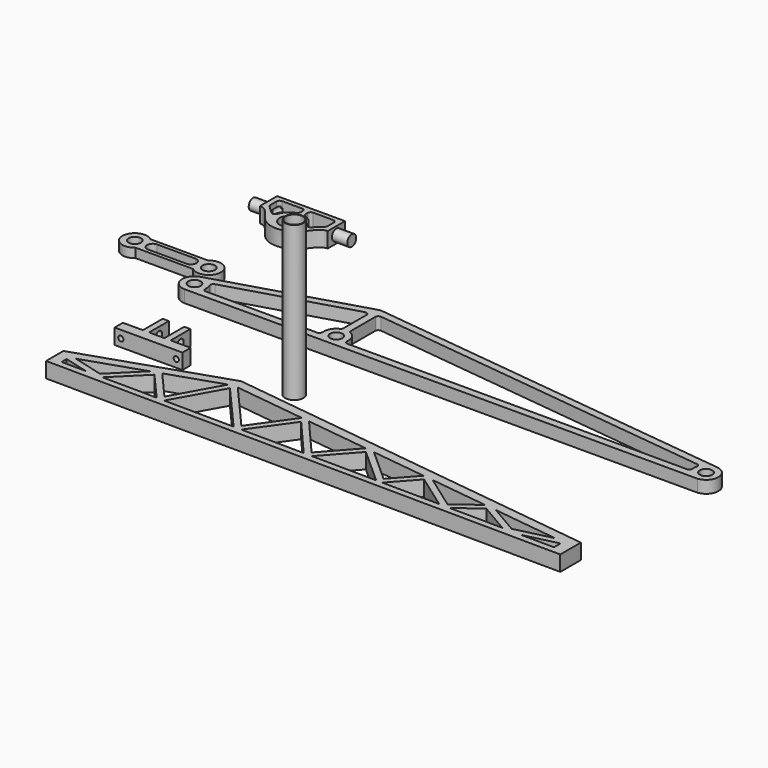
from build123d import *

# Parameters (mm, degrees)
F0_R      = 10
F1_DEPTH  = 20
F2_R      = 5
F3_R      = 10
F4_DEPTH  = 15
F5_R      = 15
F6_DEPTH  = 25
F7_R      = 9
F8_DEPTH  = 25
F13_DEPTH = 25
F14_R     = 6.3615606468
F15_DEPTH = 238.9008327255
F16_R     = 4.25
F17_DEPTH = 16.7239428354
F18_R     = 4.5979762067
F19_DEPTH = 20
F21_R     = 15
F21_R_2   = 14
F22_DEPTH = 250
F24_DEPTH = 25


# Not quite as in the source:
# - a feature of the source that left no trace in its solid (it failed there, or was rolled back) is left out
# - a pattern or mirror of a feature is missing from the dataset's text; its kind, count and spacing are read off the source's solid


with BuildPart() as f1:
    # F0 (on Top) → F1 (new body)
    with BuildSketch(Plane.XY):
        with BuildLine():
            Line((567.1867912898, 20), (-31.031592147, 89.5228215324))
            ThreePointArc((-31.031592147, 89.5228215324), (-35.1003415232, 89.5789443296), (-39.0962379428, 88.81038525))
            Line((-39.0962379428, 88.81038525), (-270.8933937767, 19.1538539919))
            ThreePointArc((-270.8933937767, 19.1538539919), (-284.9248706815, -2.9088588966), (-265.1375378668, -20))
            Line((-265.1375378668, -20), (567.1867912898, -20))
            ThreePointArc((567.1867912898, -20), (584.9970717899, 0), (567.1867912898, 20))
        make_face()
        with Locations((-265.1375378668, 0)):
            Circle(F0_R, mode=Mode.SUBTRACT)
        with Locations((-35.1375378668, 0)):
            Circle(F0_R, mode=Mode.SUBTRACT)
        with BuildLine():
            ThreePointArc((-246.807235087, -8), (-245.3502050521, 2.9088588966), (-249.8850830771, 12.936870676))
            Line((-249.8850830771, 12.936870676), (-41.1375378668, 75.6668461828))
            Line((-41.1375378668, 75.6668461828), (-41.1375378668, 19.0787840283))
            ThreePointArc((-41.1375378668, 19.0787840283), (-53.3393521844, 8.2881816792), (-53.4678406467, -8))
            Line((-53.4678406467, -8), (-246.807235087, -8))
        make_face(mode=Mode.SUBTRACT)
        with Locations((564.8624621332, 0)):
            Circle(F0_R, mode=Mode.SUBTRACT)
        with BuildLine():
            ThreePointArc((-16.807235087, -8), (-16.9357235492, 8.2881816792), (-29.1375378668, 19.0787840283))
            Line((-29.1375378668, 19.0787840283), (-29.1375378668, 77.221935459))
            Line((-29.1375378668, 77.221935459), (547.6527036309, 10.1894166807))
            ThreePointArc((547.6527036309, 10.1894166807), (544.9003052161, 1.2297525035), (546.5321593533, -8))
            Line((546.5321593533, -8), (-16.807235087, -8))
        make_face(mode=Mode.SUBTRACT)
    extrude(amount=F1_DEPTH)

    # F2
    f2_edges = [f1.edges().sort_by_distance(p)[0] for p in [
        (547.652704, 10.189417, 10),
        (546.532159, -8, 10),
        (-29.137538, 77.221935, 10),
        (-29.137538, 19.078784, 10),
        (-16.807235, -8, 10),
        (-53.467841, -8, 10),
        (-41.137538, 19.078784, 10),
        (-41.137538, 75.666846, 10),
        (-246.807235, -8, 10),
        (-249.885083, 12.936871, 10),
    ]]
    fillet(f2_edges, radius=F2_R)


with BuildPart() as f4:
    # F3 (on Top) → F4 (new body)
    with BuildSketch(Plane.XY):
        with BuildLine():
            Line((-297.414090761, 67.674737215), (-390.9565776503, 67.674737215))
            ThreePointArc((-390.9565776503, 67.674737215), (-424.1853342056, 52.674737215), (-390.9565776503, 37.674737215))
            Line((-390.9565776503, 37.674737215), (-297.414090761, 37.674737215))
            ThreePointArc((-297.414090761, 37.674737215), (-264.1853342056, 52.674737215), (-297.414090761, 67.674737215))
        make_face()
        with Locations((-404.1853342056, 52.674737215)):
            Circle(F3_R, mode=Mode.SUBTRACT)
        with Locations((-284.1853342056, 52.674737215)):
            Circle(F3_R, mode=Mode.SUBTRACT)
        with BuildLine():
            ThreePointArc((-375.1853342056, 43.674737215), (-384.1853342056, 52.674737215), (-375.1853342056, 61.674737215))
            Line((-375.1853342056, 61.674737215), (-313.1853342056, 61.674737215))
            ThreePointArc((-313.1853342056, 61.674737215), (-304.1853342056, 52.674737215), (-313.1853342056, 43.674737215))
            Line((-313.1853342056, 43.674737215), (-375.1853342056, 43.674737215))
        make_face(mode=Mode.SUBTRACT)
    extrude(amount=F4_DEPTH)


with BuildPart() as f6:
    # F5 (on Top) → F6 (new body)
    with BuildSketch(Plane.XY):
        with BuildLine():
            Line((-217.3005115986, 245.3892374753), (-327.3005115986, 245.3892374753))
            Line((-327.3005115986, 245.3892374753), (-327.3005115986, 210.3892374753))
            add(Edge.make_bspline(
                [(-327.3005115986, 210.3892374753), (-307.3005115986, 210.3892374753), (-307.3005115986, 175.3892374753), (-272.3005115986, 175.3892374753)],
                knots=[0, 0, 0, 0, 65.192024052, 65.192024052, 65.192024052, 65.192024052], degree=3))
            add(Edge.make_bspline(
                [(-217.3005115986, 210.3892374753), (-237.3005115986, 210.3892374753), (-237.3005115986, 175.3892374753), (-272.3005115986, 175.3892374753)],
                knots=[0, 0, 0, 0, 65.192024052, 65.192024052, 65.192024052, 65.192024052], degree=3))
            Line((-217.3005115986, 210.3892374753), (-217.3005115986, 245.3892374753))
        make_face()
        with Locations((-272.3005115986, 200.3892374753)):
            Circle(F5_R, mode=Mode.SUBTRACT)
        with BuildLine():
            Line((-313.7724625721, 238.4117428172), (-281.3005115986, 238.4117428172))
            ThreePointArc((-281.3005115986, 238.4117428172), (-277.7649776927, 236.9472767232), (-276.3005115986, 233.4117428172))
            Line((-276.3005115986, 233.4117428172), (-276.3005115986, 229.7345567962))
            ThreePointArc((-276.3005115986, 229.7345567962), (-277.4218413879, 226.2407813042), (-280.3669495445, 224.0521320333))
            ThreePointArc((-280.3669495445, 224.0521320333), (-290.3349269514, 217.7028120017), (-296.2725894189, 207.4842698908))
            ThreePointArc((-296.2725894189, 207.4842698908), (-299.7611526365, 204.0768129016), (-304.4918862976, 205.2604494523))
            Line((-304.4918862976, 205.2604494523), (-317.1973438867, 217.2057560035))
            ThreePointArc((-317.1973438867, 217.2057560035), (-318.3618201836, 218.8641946784), (-318.7724625721, 220.848582925))
            Line((-318.7724625721, 220.848582925), (-318.7724625721, 233.4117428172))
            ThreePointArc((-318.7724625721, 233.4117428172), (-317.307996478, 236.9472767232), (-313.7724625721, 238.4117428172))
        make_face(mode=Mode.SUBTRACT)
        with BuildLine():
            ThreePointArc((-248.3284337783, 207.4842698908), (-254.2660962457, 217.7028120017), (-264.2340736527, 224.0521320333))
            ThreePointArc((-264.2340736527, 224.0521320333), (-267.1791818093, 226.2407813042), (-268.3005115986, 229.7345567962))
            Line((-268.3005115986, 229.7345567962), (-268.3005115986, 233.4117428172))
            ThreePointArc((-268.3005115986, 233.4117428172), (-266.8360455045, 236.9472767232), (-263.3005115986, 238.4117428172))
            Line((-263.3005115986, 238.4117428172), (-230.8285606251, 238.4117428172))
            ThreePointArc((-230.8285606251, 238.4117428172), (-227.2930267191, 236.9472767232), (-225.8285606251, 233.4117428172))
            Line((-225.8285606251, 233.4117428172), (-225.8285606251, 220.848582925))
            ThreePointArc((-225.8285606251, 220.848582925), (-226.2392030135, 218.8641946784), (-227.4036793104, 217.2057560035))
            Line((-227.4036793104, 217.2057560035), (-240.1091368996, 205.2604494523))
            ThreePointArc((-240.1091368996, 205.2604494523), (-244.8398705607, 204.0768129016), (-248.3284337783, 207.4842698908))
        make_face(mode=Mode.SUBTRACT)
    extrude(amount=F6_DEPTH)

    # F7 (on face) → F8 (join)
    with BuildSketch(Plane(origin=(-327.3005115986, 0, 0), x_dir=(0, -1, 0), z_dir=(-1, 0, 0))):
        with Locations((-227.8892374753, 12.5)):
            Circle(F7_R)
    f8 = extrude(amount=F8_DEPTH)

    # F8_copies: F8 across plane
    add(f8.mirror(Plane(origin=(-272.300512, 0, 0), x_dir=(0, 0, 1), z_dir=(1, 0, 0))))

    # F18 (on face) → F19 (cut)
    with BuildSketch(Plane(origin=(0, 245.3892374753, 0), x_dir=(-1, 0, 0), z_dir=(0, 1, 0))):
        with Locations((317.3005115986, 12.5)):
            Circle(F18_R)
        with Locations((227.3005115986, 12.5)):
            Circle(F18_R)
    extrude(amount=-F19_DEPTH, mode=Mode.SUBTRACT)


with BuildPart() as f13:
    # F12 (on Top) → F13 (new body)
    with BuildSketch(Plane.XY):
        Polygon((-262.7855014801, -148.1870505672), (-262.7855014801, -164.9099934026), (-207.7855014801, -164.9099934026), (-207.7855014801, -148.1870505672), (-220.2855014801, -148.1870505672), (-220.2855014801, -108.1870505672), (-230.2855014801, -108.1870505672), (-230.2855014801, -148.1870505672), align=None)
        Polygon((-207.7855014801, -148.1870505672), (-207.7855014801, -164.9099934026), (-152.7855014801, -164.9099934026), (-152.7855014801, -148.1870505672), (-185.2855014801, -148.1870505672), (-185.2855014801, -108.1870505672), (-195.2855014801, -108.1870505672), (-195.2855014801, -148.1870505672), align=None)
    extrude(amount=F13_DEPTH)

    # F14 (on face) → F15 (cut, through all)
    with BuildSketch(Plane.YZ.offset(-185.2855014801)):
        with Locations((-128.1870505672, 12.5)):
            Circle(F14_R)
    extrude(amount=-F15_DEPTH, mode=Mode.SUBTRACT)

    # F16 (on face) → F17 (cut, through all)
    with BuildSketch(Plane(origin=(0, -148.1870505672, 0), x_dir=(-1, 0, 0), z_dir=(0, 1, 0))):
        with Locations((162.7855014801, 12.5)):
            Circle(F16_R)
        with Locations((252.7855014801, 12.5)):
            Circle(F16_R)
    extrude(amount=-F17_DEPTH, mode=Mode.SUBTRACT)


with BuildPart() as f22:
    # F21 (on Top) → F22 (new body)
    with BuildSketch(Plane.XY):
        with Locations((0, -129.0528408765)):
            Circle(F21_R)
        with Locations((0, -129.0528408765)):
            Circle(F21_R_2, mode=Mode.SUBTRACT)
    extrude(amount=F22_DEPTH)


with BuildPart() as f24:
    # F23 (on Top) → F24 (new body)
    with BuildSketch(Plane.XY):
        Polygon((-45.6561110914, -179.8242628575), (-273.2936190678, -255.6992598235), (-273.2936190678, -290.8384732402), (567.017018795, -298.4088398829), (567.017018795, -256.6455006599), align=None)
        Polygon((-216.4749437332, -281.0517338258), (-256.2147935359, -280.6937171356), (-256.2147935359, -270.3590121979), align=None, mode=Mode.SUBTRACT)
        Polygon((-189.5394681398, -281.2943957853), (-142.5139620191, -234.5043431103), (-100.9064132084, -282.0928918321), align=None, mode=Mode.SUBTRACT)
        Polygon((-198.048490499, -275.6540426765), (-247.6192130188, -262.3161478574), (-152.9199574694, -230.7514650801), align=None, mode=Mode.SUBTRACT)
        Polygon((-88.5170655798, -282.2045075845), (-44.7451068651, -203.6370840889), (24.8407358138, -283.2257491107), align=None, mode=Mode.SUBTRACT)
        Polygon((37.6322929275, -283.3409883722), (83.2624414993, -219.2051047713), (139.4630344229, -284.2583825046), align=None, mode=Mode.SUBTRACT)
        Polygon((192.6491125209, -224.8791896426), (146.1901360386, -276.7485657618), (90.2915659025, -212.0448852704), align=None, mode=Mode.SUBTRACT)
        Polygon((464.0936290162, -287.1829826629), (377.8272343086, -286.4058078808), (415.3261635857, -258.7359073498), align=None, mode=Mode.SUBTRACT)
        Polygon((494.8733425929, -287.4602773994), (548.4594728858, -274.6344028454), (548.4594728858, -287.9430353641), align=None, mode=Mode.SUBTRACT)
        Polygon((152.7810257053, -284.3783644165), (199.0722795025, -232.6962431983), (257.8296595944, -285.3247485726), align=None, mode=Mode.SUBTRACT)
        Polygon((267.8531632296, -285.4150504136), (303.7064629938, -245.3864395531), (360.8069589392, -286.2524720558), align=None, mode=Mode.SUBTRACT)
        Polygon((296.9373836381, -237.9555817425), (262.659177735, -276.2256705242), (207.3977704345, -226.7284794214), align=None, mode=Mode.SUBTRACT)
        Polygon((369.4627686999, -280.1501376635), (313.3881203593, -240.0182900547), (407.8062035951, -251.8570890346), align=None, mode=Mode.SUBTRACT)
        Polygon((474.9593976915, -281.9442413844), (427.6446621433, -254.3445735797), (534.3637862, -267.7257630057), align=None, mode=Mode.SUBTRACT)
        Polygon((-52.6849719775, -197.3416404528), (-95.1230948012, -273.5149273278), (-137.117258646, -225.4841884527), align=None, mode=Mode.SUBTRACT)
        Polygon((31.1315588838, -275.2282420249), (-38.1967581359, -195.9341214482), (77.2476430524, -210.4093470849), align=None, mode=Mode.SUBTRACT)
    extrude(amount=F24_DEPTH)


solid = Compound([f1.part, f4.part, f6.part, f13.part, f22.part, f24.part])
